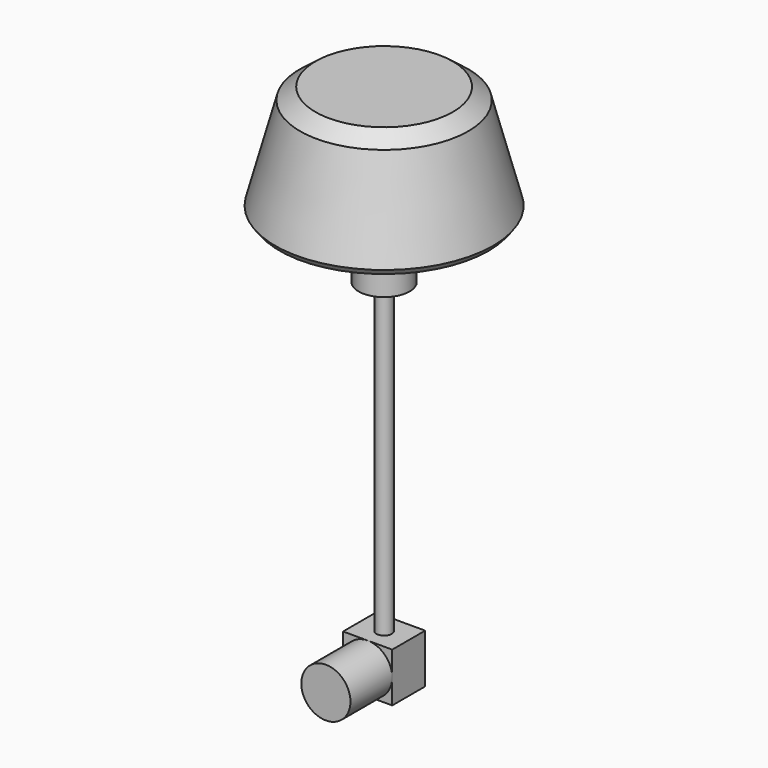
from build123d import *

# Parameters (mm, degrees)
F0_R     = 4
F1_DEPTH = 4.25
F2_W     = 8
F2_H     = 8
F3_DEPTH = 6.7
F4_R     = 1.25
F5_DEPTH = 50
F6_R     = 4.15
F7_DEPTH = 10
F8_R     = 18
F8_R_2   = 4.15
F9_DEPTH = 18
F9_TAPER = 15


# Not quite as in the source:
# - a fillet or chamfer that OpenCascade refuses, or shapes differently, is made with other operations: its cross-section is extruded or revolved along the edge and cut away or added


with BuildPart() as f1:
    # F0 (on Front) → F1 (new body, symmetric)
    with BuildSketch(Plane.XZ):
        Circle(F0_R)
    extrude(amount=F1_DEPTH, both=True)

    # F2 (on face) → F3 (join)
    with BuildSketch(Plane(origin=(0, 4.25, 0), x_dir=(-1, 0, 0), z_dir=(0, 1, 0))):
        Rectangle(F2_W, F2_H)
    extrude(amount=F3_DEPTH)

    # F4 (on face) → F5 (join)
    with BuildSketch(Plane.XY.offset(4)):
        with Locations((0, 7.6)):
            Circle(F4_R)
    extrude(amount=F5_DEPTH)

    # F6 (on face) → F7 (join)
    with BuildSketch(Plane.XY.offset(54)):
        with Locations((0, 7.6)):
            Circle(F6_R)
    extrude(amount=F7_DEPTH)

    # F8 (on face) → F9 (join)
    with BuildSketch(Plane.XY.offset(64)):
        with Locations((0, 7.6)):
            Circle(F8_R)
        with Locations((0, 7.6)):
            Circle(F8_R_2, mode=Mode.SUBTRACT)
        with Locations((0, 7.6)):
            Circle(F8_R_2)
    extrude(amount=F9_DEPTH, taper=F9_TAPER)

    # F10: chamfer of 1 on 1 edges, made by hand

    # F10_s1 → F10_t2 (revolve, cut)
    with BuildSketch(Plane.XZ.offset(-7.6)):
        Polygon((17, 64), (17.7411809549, 64.9659258263), (18, 64), align=None)
    revolve(axis=Axis((0, 7.6, 64), (0, 0, -1)), mode=Mode.SUBTRACT)

    # F11: chamfer of 2 on 1 edges, made by hand

    # F11_s1 → F11_t2 (revolve, cut)
    with BuildSketch(Plane.XZ.offset(-7.6)):
        Polygon((13.6945526264, 80.0681483474), (11.1769145362, 82), (13.1769145362, 82), align=None)
    revolve(axis=Axis((0, 7.6, 82), (0, 0, -1)), mode=Mode.SUBTRACT)


solid = f1.part
